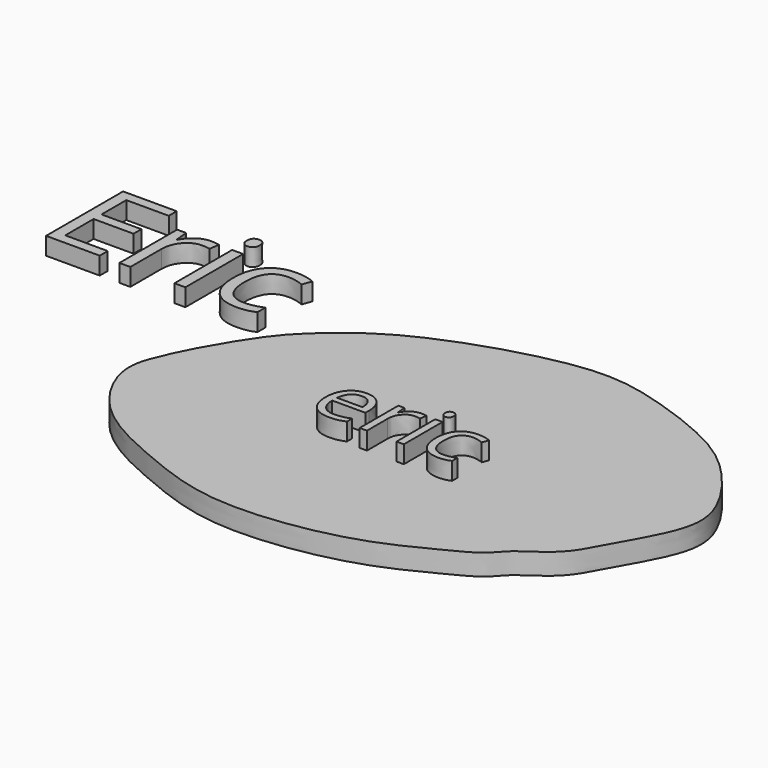
from build123d import *

# Parameters (mm, degrees)
F1_DEPTH       = 3
F2_TEXT_SIZE   = 19.186411622
F2_TEXT_SIZE_2 = 12.8528206713
F3_DEPTH       = 2.5


# Not quite as in the source:
# - Text() gives the source's letters only with a copy of the font that has no kerning and outlines rounded to 1/6400 em; it was checked with that copy


with BuildPart() as f1:
    # F0 (on Top) → F1 (new body)
    with BuildSketch(Plane.XY):
        with BuildLine():
            add(Edge.make_bspline(
                [(22.1915399245, 30.4195880448), (21.9890839131, 32.2780972423), (23.1108105918, 35.3006306033), (25.1213549482, 39.620762313), (29.5692654213, 47.0808967164), (33.7900012294, 51.1764710634), (41.6686183411, 57.4933860799), (61.601683858, 63.7738325209), (71.9083542332, 62.0594423574), (83.9169139579, 57.571702408), (89.4119687301, 52.7987211895), (93.558787577, 47.3988056457), (96.0542597753, 40.7713888706), (90.5964445628, 31.9030907701), (87.9377882596, 26.168929737), (82.7109481272, 23.3313216329), (81.2533983532, 20.8251033587), (75.9355984287, 18.2205575494), (70.2927905901, 15.2710404976), (61.1834480536, 12.6299252405), (48.0305585041, 11.614909374), (37.160227335, 15.9306380707), (26.234907204, 20.879109721), (22.4743649638, 27.8233058525), (22.1915399245, 30.4195880448)],
                knots=[0, 0, 0, 0, 0.0348874191, 0.0697619895, 0.1157845056, 0.1538223092, 0.2037358259, 0.2751568718, 0.3273394434, 0.3826702248, 0.4253025964, 0.4658341742, 0.5060714709, 0.5557709574, 0.5963173342, 0.6329752135, 0.6594590188, 0.6966754995, 0.7369449094, 0.7854468549, 0.8424311254, 0.8966096497, 0.951263311, 1, 1, 1, 1], degree=3))
        make_face()
    extrude(amount=F1_DEPTH)

    # F2 (on face) → F3 (join)
    with BuildSketch(Plane.XY.offset(3)):
        with Locations((-3.6818312398, 46.3618335056)):
            Text('Eric', F2_TEXT_SIZE, font='Open Sans', text_align=(TextAlign.LEFT, TextAlign.BOTTOM))
        with Locations((45.9847450256, 32.0262089372)):
            Text('eric', F2_TEXT_SIZE_2, font='Open Sans', text_align=(TextAlign.LEFT, TextAlign.BOTTOM))
    extrude(amount=F3_DEPTH)


solid = f1.part
